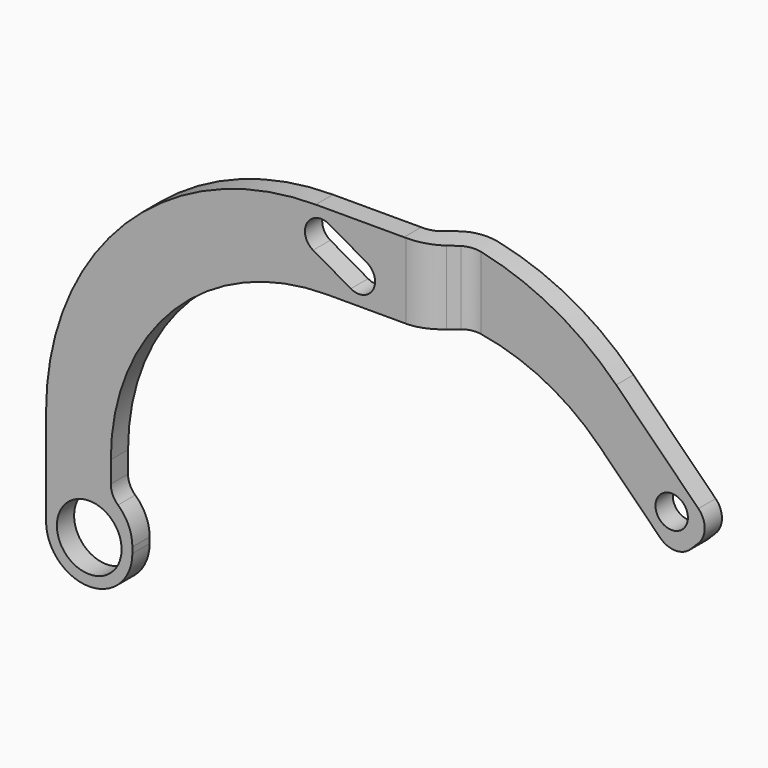
from build123d import *

# Parameters (mm, degrees)
F0_R        = 3
F0_R_2      = 1.5
F1_DEPTH    = 4.5
F2_R        = 20
F3_R        = 25
F4_R        = 25
F5_T1_DEPTH = 24.5
F5_T3_DEPTH = 21.8205080757
F6_R        = 2
F8_DEPTH    = 50
F9_R        = 2
F10_R       = 4


# Not quite as in the source:
# - a fillet or chamfer that OpenCascade refuses, or shapes differently, is made with other operations: its cross-section is extruded or revolved along the edge and cut away or added
# - a feature names something its author has since deleted; it is built from what else it names


with BuildPart() as f1:
    # F0 (on Front) → F1 (new body)
    with BuildSketch(Plane.XZ):
        Polygon((-4, 27), (-4, -4), (4, -4), (4, 4), (2, 4), (2, 27), align=None)
        Circle(F0_R, mode=Mode.SUBTRACT)
        Polygon((-4, 34), (-4, 27), (2, 27), (4, 27), (39.4644660941, 27), (52.3535533906, 14.1109127035), (55.8890872965, 17.6464466094), (39.5355339059, 34), align=None)
        with BuildLine():
            ThreePointArc((25.7442084075, 30.8023647132), (26.3023647132, 28.7557915925), (24.2557915925, 28.1976352868))
            Line((24.2557915925, 28.1976352868), (20.7557915925, 30.1976352868))
            ThreePointArc((20.7557915925, 30.1976352868), (20.1976352868, 32.2442084075), (22.2442084075, 32.8023647132))
            Line((22.2442084075, 32.8023647132), (25.7442084075, 30.8023647132))
        make_face(mode=Mode.SUBTRACT)
        with Locations((52, 18)):
            Circle(F0_R_2, mode=Mode.SUBTRACT)
    extrude(amount=F1_DEPTH)

    # F2
    f2_edges = [f1.edges().sort_by_distance(p)[0] for p in [
        (39.464466, -2.25, 27),
        (2, -2.25, 27),
    ]]
    fillet(f2_edges, radius=F2_R)

    # F3
    f3_edges = [f1.edges().sort_by_distance(p)[0] for p in [
        (-4, -2.25, 34),
    ]]
    fillet(f3_edges, radius=F3_R)

    # F4
    f4_edges = [f1.edges().sort_by_distance(p)[0] for p in [
        (39.535534, -2.25, 34),
    ]]
    fillet(f4_edges, radius=F4_R)

    # F5: fillet of radius 4 on 3 edges, made by hand

    # F5_s2 → F5_t1 (cut)
    with BuildSketch(Plane.XZ.offset(-10)):
        with BuildLine():
            ThreePointArc((0, -4), (2.8284271247, -2.8284271247), (4, 0))
            Line((4, 0), (4, -4))
            Line((4, -4), (0, -4))
        make_face()
        with BuildLine():
            ThreePointArc((-4, 0), (-2.8284271247, -2.8284271247), (0, -4))
            Line((0, -4), (-4, -4))
            Line((-4, -4), (-4, 0))
        make_face()
    extrude(amount=F5_T1_DEPTH, mode=Mode.SUBTRACT)

    # F5_s4 → F5_t3 (cut)
    with BuildSketch(Plane.XZ.offset(-8.6602540378)):
        with BuildLine():
            ThreePointArc((4, 0.5358983849), (3.4641016151, 2.5358983849), (2, 4))
            Line((2, 4), (4, 4))
            Line((4, 4), (4, 0.5358983849))
        make_face()
    extrude(amount=F5_T3_DEPTH, mode=Mode.SUBTRACT)

    # F6
    f6_edges = [f1.edges().sort_by_distance(p)[0] for p in [
        (2, -2.25, 4),
        (52.353553, -2.25, 14.110913),
        (55.889087, -2.25, 17.646447),
    ]]
    fillet(f6_edges, radius=F6_R)

    # F7 (on Top) → F8 (cut, symmetric)
    with BuildSketch(Plane.XY):
        Polygon((34.1801948466, 1.5), (-25.8198051534, 1.5), (-25.8198051534, -2.5), (30.1801948466, -2.5), align=None)
        Polygon((33.5086219714, -2), (29.5086219714, -6), (69.5086219714, -6), (69.5086219714, -2), align=None)
    extrude(amount=F8_DEPTH, both=True, mode=Mode.SUBTRACT)

    # F9
    f9_edges = [f1.edges().sort_by_distance(p)[0] for p in [
        (33.508622, -2, 30.243221),
        (30.180195, -2.5, 30.489996),
    ]]
    fillet(f9_edges, radius=F9_R)

    # F10
    f10_edges = [f1.edges().sort_by_distance(p)[0] for p in [
        (31.008622, -4.5, 30.466524),
        (32.680195, 0, 30.348729),
    ]]
    fillet(f10_edges, radius=F10_R)


solid = f1.part
